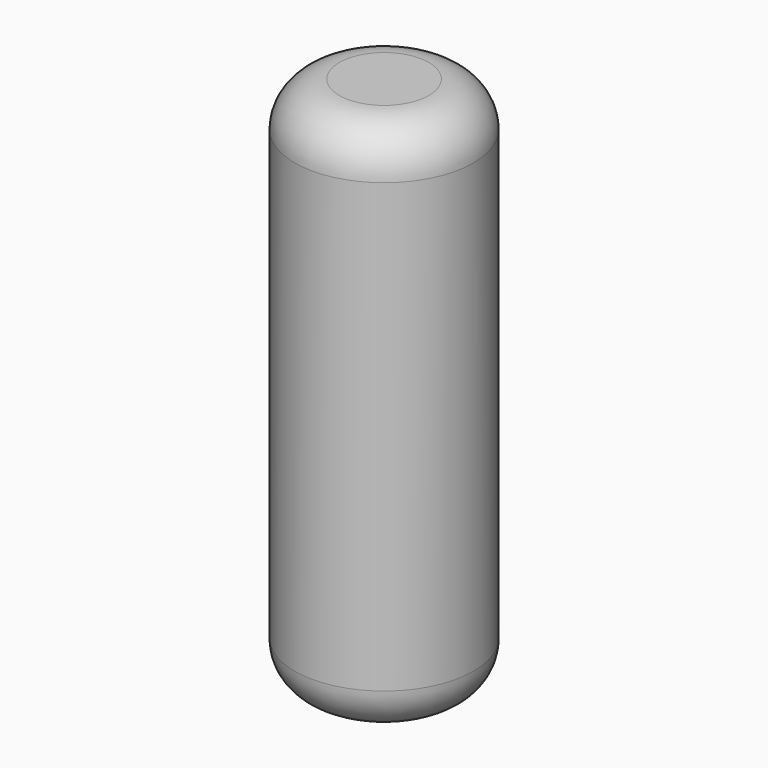
from build123d import *

# Parameters (mm, degrees)
F0_R     = 10
F1_DEPTH = 30
F2_R     = 5
F3_R     = 5
F4_T     = -2.5


# Not quite as in the source:
# - the program builds the solid bodies; features that only make, move or delete a surface that nothing else refers to are left out


with BuildPart() as f1:
    # F0 (on Top) → F1 (new body, symmetric)
    with BuildSketch(Plane.XY):
        with Locations((-2.7793468907, 0.249794306)):
            Circle(F0_R)
    extrude(amount=F1_DEPTH, both=True)

    # F2
    f2_edges = [f1.edges().sort_by_distance(p)[0] for p in [
        (-12.779347, 0.249794, 30),
    ]]
    fillet(f2_edges, radius=F2_R)

    # F3
    f3_edges = [f1.edges().sort_by_distance(p)[0] for p in [
        (-12.779347, 0.249794, -30),
    ]]
    fillet(f3_edges, radius=F3_R)

    # F4 (hollow: no face is removed)
    offset(amount=F4_T, mode=Mode.SUBTRACT)


solid = f1.part
